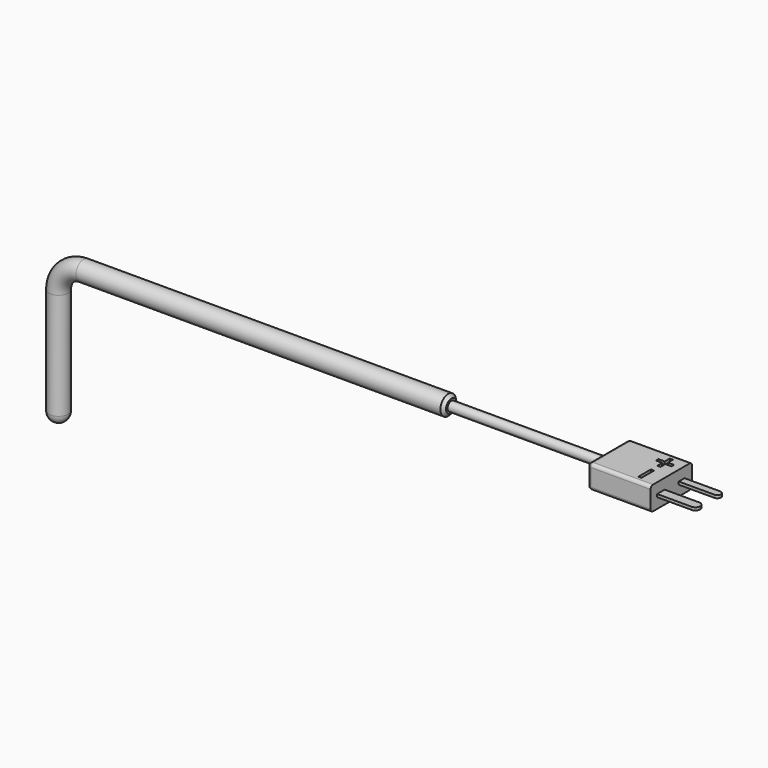
from build123d import *

# Parameters (mm, degrees)
F1_R      = 3.1
F3_R      = 3.1
F4_R      = 1.5
F5_DEPTH  = 50
F6_SIZE   = 1
F7_W      = 16.5
F7_H      = 7.5
F7_R      = 1.5
F8_DEPTH  = 20
F9_W      = 3
F9_H      = 0.9
F10_DEPTH = 12.5
F9_W_2    = 2.3
F11_R     = 1
F12_R     = 1.49999
F13_R     = 1.14999
F14_W     = 1
F14_H     = 5
F14_H_2   = 2
F14_W_2   = 2
F14_H_3   = 1
F15_DEPTH = 1


# Not quite as in the source:
# - a fillet or chamfer is up to 0.001 mm smaller than in the source, because OpenCascade refuses the exact size


with BuildPart() as f2:
    # F2: sweep along a path in F0
    with BuildLine(Plane.XZ) as f2_path:
        Line((0, 0), (0, 37))
        ThreePointArc((0, 37), (2.3431457505, 42.6568542495), (8, 45))
        Line((8, 45), (125, 45))
    # F1 (on Top) → F2 (sweep)
    with BuildSketch(Plane.XY):
        Circle(F1_R)
    sweep(path=f2_path.line)

    # F3
    f3_edges = [f2.edges().sort_by_distance(p)[0] for p in [
        (-3.1, 0, 0),
    ]]
    fillet(f3_edges, radius=F3_R)

    # F6
    f6_edges = [f2.edges().sort_by_distance(p)[0] for p in [
        (125, 0, 48.1),
    ]]
    chamfer(f6_edges, length=F6_SIZE)


with BuildPart() as f5:
    # F4 (on face) → F5 (new body)
    with BuildSketch(Plane.YZ.offset(125)):
        with Locations((0, 45)):
            Circle(F4_R)
    extrude(amount=F5_DEPTH)

    # F7 (on face) → F8 (join)
    with BuildSketch(Plane.YZ.offset(175)):
        with Locations((0, 45)):
            Rectangle(F7_W, F7_H)
        with Locations((0, 45)):
            Circle(F7_R, mode=Mode.SUBTRACT)
        with Locations((0, 45)):
            Circle(F7_R)
    extrude(amount=F8_DEPTH)

    # F11
    f11_edges = [f5.edges().sort_by_distance(p)[0] for p in [
        (185, -8.25, 48.75),
        (175, 0, 48.75),
        (185, 8.25, 48.75),
        (175, 8.25, 45),
        (185, 8.25, 41.25),
        (175, 0, 41.25),
        (185, -8.25, 41.25),
        (175, -8.25, 45),
    ]]
    fillet(f11_edges, radius=F11_R)

    # F14 (on face) → F15 (cut)
    with BuildSketch(Plane.XY.offset(48.75)):
        with Locations((190, -3.75)):
            Rectangle(F14_W, F14_H)
        with Locations((190, 5.25)):
            Rectangle(F14_W, F14_H_2)
        with Locations((191.5, 3.75)):
            Rectangle(F14_W_2, F14_H_3)
        with Locations((190, 3.75)):
            Rectangle(F14_W, F14_H_3)
        with Locations((190, 2.25)):
            Rectangle(F14_W, F14_H_2)
        with Locations((188.5, 3.75)):
            Rectangle(F14_W_2, F14_H_3)
    extrude(amount=-F15_DEPTH, mode=Mode.SUBTRACT)


with BuildPart() as f10:
    # F9 (on face) → F10 (new body)
    with BuildSketch(Plane.YZ.offset(195)):
        with Locations((-4.15, 45)):
            Rectangle(F9_W, F9_H)
    extrude(amount=F10_DEPTH)

    # F12 (radius 1.5 in the source; OpenCascade refuses exactly that, so slightly less here)
    f12_edges = [f10.edges().sort_by_distance(p)[0] for p in [
        (207.5, -2.65, 45),
        (207.5, -5.65, 45),
    ]]
    fillet(f12_edges, radius=F12_R)


with BuildPart() as f10b:
    # F9 (on face) → F10, piece 2 (new body)
    with BuildSketch(Plane.YZ.offset(195)):
        with Locations((4.1, 45)):
            Rectangle(F9_W_2, F9_H)
    extrude(amount=F10_DEPTH)

    # F13 (radius 1.15 in the source; OpenCascade refuses exactly that, so slightly less here)
    f13_edges = [f10b.edges().sort_by_distance(p)[0] for p in [
        (207.5, 5.25, 45),
        (207.5, 2.95, 45),
    ]]
    fillet(f13_edges, radius=F13_R)


solid = Compound([f2.part, f5.part, f10.part, f10b.part])
